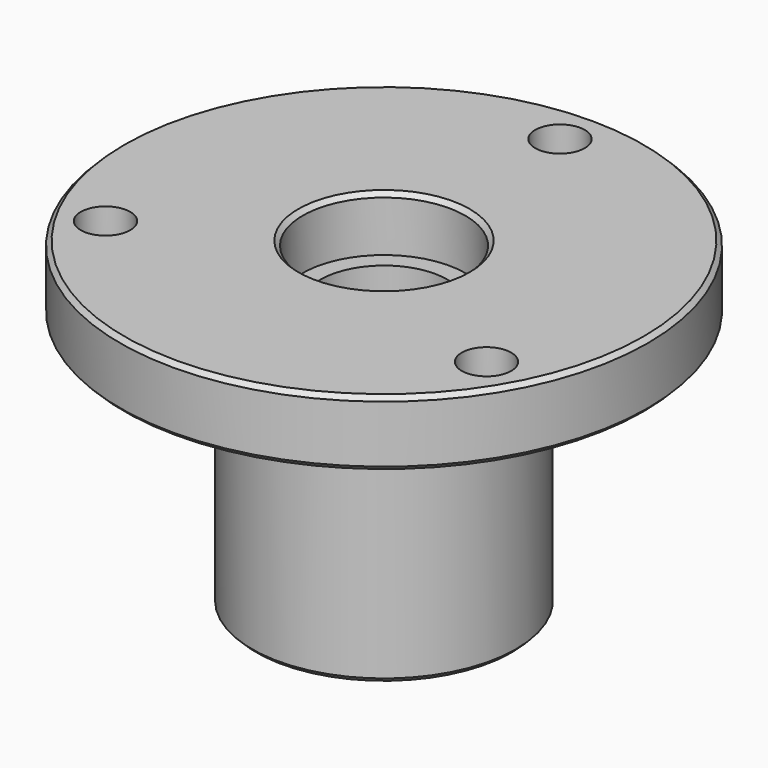
from build123d import *

# Parameters (mm, degrees)
F0_R           = 30
F1_DEPTH       = 58
F2_R           = 60
F2_R_2         = 30
F3_DEPTH       = 15
F4_R           = 18.475
F5_DEPTH       = 12.5
F6_D           = 6.6
F6_CBORE_D     = 11.25
F6_CBORE_DEPTH = 6
F7_R           = 20.975
F8_DEPTH       = 12
F10_D          = 28.9
F11_SIZE       = 1


# Not quite as in the source:
# - a feature names something its author has since deleted; it is built from what else it names


with BuildPart() as f1:
    # F0 (on Top) → F1 (new body)
    with BuildSketch(Plane.XY):
        Circle(F0_R)
    extrude(amount=F1_DEPTH)

    # F2 (on face) → F3 (join)
    with BuildSketch(Plane.XY.offset(58)):
        Circle(F2_R)
        Circle(F2_R_2, mode=Mode.SUBTRACT)
        Circle(F2_R_2)
    extrude(amount=F3_DEPTH)

    # F4 (on face) → F5 (cut)
    with BuildSketch(Plane.XY.offset(73)):
        Circle(F4_R)
    extrude(amount=-F5_DEPTH, mode=Mode.SUBTRACT)

    # F6 (through all)
    with Locations(Plane.XY.offset(73)):
        with Locations((-43.3012701892, -25), (0, 50), (43.3012701892, -25)):
            CounterBoreHole(F6_D / 2, F6_CBORE_D / 2, F6_CBORE_DEPTH)

    # F7 (on face) → F8 (cut)
    with BuildSketch(Plane(origin=(0, 0, 0), x_dir=(1, 0, 0), z_dir=(0, 0, -1))):
        Circle(F7_R)
    extrude(amount=-F8_DEPTH, mode=Mode.SUBTRACT)

    # F10 (through all)
    with Locations(Plane.XY.offset(73)):
        with Locations((0, 0)):
            Hole(F10_D / 2)

    # F11
    f11_edges = [f1.edges().sort_by_distance(p)[0] for p in [
        (-60, 0, 73),
        (-60, 0, 58),
        (-30, 0, 0),
        (-20.975, 0, 0),
        (-18.475, 0, 73),
    ]]
    chamfer(f11_edges, length=F11_SIZE)


solid = f1.part
